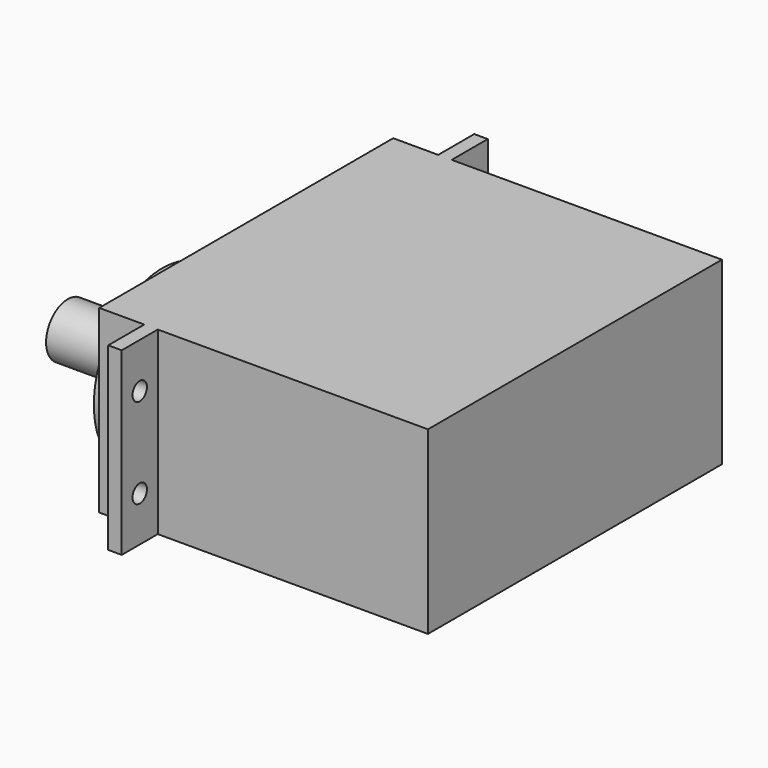
from build123d import *

# Parameters (mm, degrees)
F0_W      = 36.5
F0_H      = 20
F1_DEPTH  = 20.4
F3_W      = 5
F3_H      = 20
F4_DEPTH  = 1.5
F7_DEPTH  = 1
F8_R      = 6
F9_DEPTH  = 0.5
F10_R     = 3
F11_DEPTH = 0.5
F12_R     = 3
F13_DEPTH = 10
F14_R     = 1
F15_DEPTH = 25


# Not quite as in the source:
# - a pattern or mirror of a feature is missing from the dataset's text; its kind, count and spacing are read off the source's solid


with BuildPart() as f1:
    # F0 (on Front) → F1 (new body, symmetric)
    with BuildSketch(Plane.XZ):
        with Locations((18.25, 10)):
            Rectangle(F0_W, F0_H)
    extrude(amount=F1_DEPTH, both=True)

    # F3 (on offset) → F4 (join)
    with BuildSketch(Plane.YZ.offset(5)):
        with Locations((-22.9, 10)):
            Rectangle(F3_W, F3_H)
    extrude(amount=F4_DEPTH)


with BuildPart() as f5_1:
    # F5: instance of F1
    add(f1.part.mirror(Plane.XZ))


with BuildPart() as f1_1:
    add(f1.part)

    add(f5_1.part)  # F7 merges F5_1
    # F6 (on face) → F7 (join)
    with BuildSketch(Plane(origin=(0, 0, 0), x_dir=(0, -1, 0), z_dir=(-1, 0, 0))):
        with BuildLine():
            Line((-13.8426406871, 1.5), (6.1573593129, 1.5))
            ThreePointArc((6.1573593129, 1.5), (19.9, 10), (6.1573593129, 18.5))
            Line((6.1573593129, 18.5), (-13.8426406871, 18.5))
            Line((-13.8426406871, 18.5), (-13.8426406871, 1.5))
        make_face()
    extrude(amount=F7_DEPTH)

    # F8 (on face) → F9 (join)
    with BuildSketch(Plane(origin=(-1, 0, 0), x_dir=(0, -1, 0), z_dir=(-1, 0, 0))):
        with Locations((10.4, 10.05)):
            Circle(F8_R)
    extrude(amount=F9_DEPTH)

    # F10 (on face) → F11 (cut)
    with BuildSketch(Plane(origin=(-1.5, 0, 0), x_dir=(0, -1, 0), z_dir=(-1, 0, 0))):
        with Locations((10.4, 10.05)):
            Circle(F10_R)
    extrude(amount=-F11_DEPTH, mode=Mode.SUBTRACT)

    # F14 (on face) → F15 (cut)
    with BuildSketch(Plane(origin=(5, 0, 0), x_dir=(0, -1, 0), z_dir=(-1, 0, 0))):
        with Locations((-22.9, 5)):
            Circle(F14_R)
        with Locations((-22.9, 15)):
            Circle(F14_R)
    f15 = extrude(amount=-F15_DEPTH, mode=Mode.SUBTRACT)

    # F15_copies: F15 across plane
    add(f15.mirror(Plane(origin=(0, 0, 0), x_dir=(0, 0, -1), z_dir=(0, -1, 0))), mode=Mode.SUBTRACT)


with BuildPart() as f13:
    # F12 (on face) → F13 (new body)
    with BuildSketch(Plane(origin=(-1.5, 0, 0), x_dir=(0, -1, 0), z_dir=(-1, 0, 0))):
        with Locations((10.4, 10.05)):
            Circle(F12_R)
    extrude(amount=F13_DEPTH)


solid = Compound([f1_1.part, f13.part])
